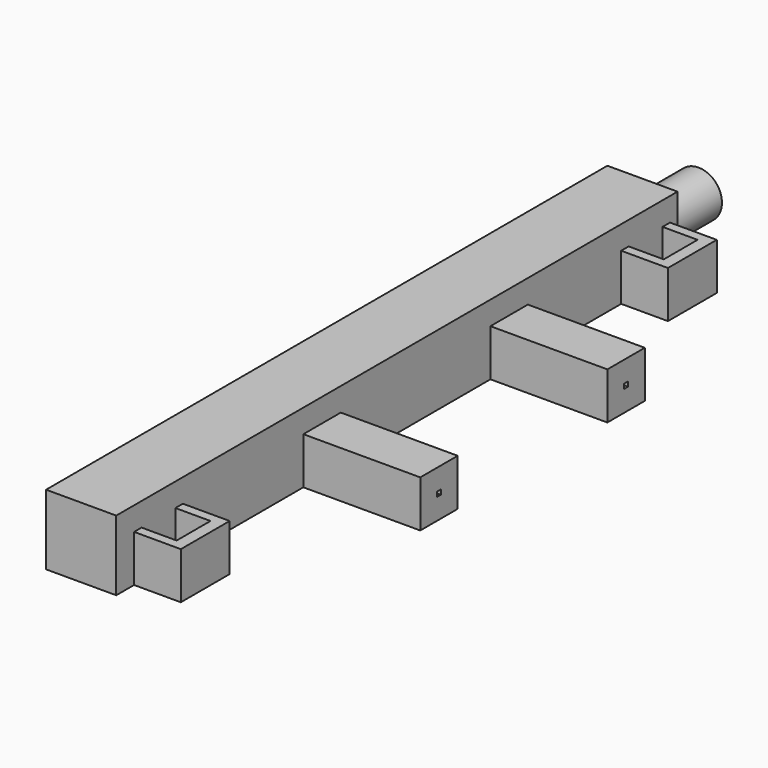
from build123d import *

# Parameters (mm, degrees)
F1_DEPTH = 15
F0_W     = 25
F0_H     = 10
F0_W_2   = 2.5
F0_H_2   = 9.0467076302
F2_DEPTH = 10
F3_W     = 4
F3_H     = 4
F4_DEPTH = 100
F6_W     = 1
F6_H     = 1
F5_W     = 1
F5_H     = 1
F7_DEPTH = 30
F8_R     = 5
F8_R_2   = 4
F9_DEPTH = 15


with BuildPart() as f1:
    # F0 (on Top) → F1 (new body)
    with BuildSketch(Plane.XY):
        Polygon((-29.806669808, 70.373563841), (-44.806669808, 70.373563841), (-44.806669808, -79.626436159), (-29.806669808, -79.626436159), (-29.806669808, -74.8653486371), (-29.806669808, -72.8653486371), (-29.806669808, -63.8186410069), (-29.806669808, -61.8186410069), (-29.806669808, -29.626436159), (-29.806669808, -19.626436159), (-29.806669808, 20.373563841), (-29.806669808, 30.373563841), (-29.806669808, 55.3112663329), (-29.806669808, 57.3112663329), (-29.806669808, 66.357973963), (-29.806669808, 68.357973963), align=None)
    extrude(amount=F1_DEPTH)

    # F0 (on Top) → F2 (join)
    with BuildSketch(Plane.XY):
        with Locations((-17.306669808, 25.373563841)):
            Rectangle(F0_W, F0_H)
        with Locations((-17.306669808, -24.626436159)):
            Rectangle(F0_W, F0_H)
        Polygon((-29.806669808, -61.8186410069), (-29.806669808, -63.8186410069), (-22.306669808, -63.8186410069), (-19.806669808, -63.8186410069), (-19.806669808, -61.8186410069), align=None)
        with Locations((-21.056669808, -68.341994822)):
            Rectangle(F0_W_2, F0_H_2)
        Polygon((-29.806669808, -72.8653486371), (-29.806669808, -74.8653486371), (-19.806669808, -74.8653486371), (-19.806669808, -72.8653486371), (-22.306669808, -72.8653486371), align=None)
        Polygon((-22.3066698015, 57.3112663329), (-29.8066698015, 57.3112663329), (-29.806669808, 55.3112663329), (-19.8066698015, 55.3112663329), (-19.8066698015, 57.3112663329), align=None)
        with Locations((-21.0566698015, 61.8346201479)):
            Rectangle(F0_W_2, F0_H_2)
        Polygon((-19.8066698015, 68.357973963), (-29.8066698015, 68.357973963), (-29.806669808, 66.357973963), (-22.3066698015, 66.357973963), (-19.8066698015, 66.357973963), align=None)
    extrude(amount=F2_DEPTH)

    # F3 (on face) → F4 (cut)
    with BuildSketch(Plane(origin=(0, 70.373563841, 0), x_dir=(-1, 0, 0), z_dir=(0, 1, 0))):
        with Locations((36.806669808, 6)):
            Rectangle(F3_W, F3_H)
    extrude(amount=-F4_DEPTH, mode=Mode.SUBTRACT)

    # F6 (on face) + F5 (on face) → F7 (cut)
    with BuildSketch(Plane.YZ.offset(-4.806669808)):
        with Locations((25.373563841, 5)):
            Rectangle(F6_W, F6_H)
    with BuildSketch(Plane.YZ.offset(-4.806669808)):
        with Locations((-24.626436159, 5)):
            Rectangle(F5_W, F5_H)
    extrude(amount=-F7_DEPTH, mode=Mode.SUBTRACT)

    # F8 (on face) → F9 (join)
    with BuildSketch(Plane(origin=(0, 70.373563841, 0), x_dir=(-1, 0, 0), z_dir=(0, 1, 0))):
        with Locations((37.306669808, 6)):
            Circle(F8_R)
        with Locations((37.306669808, 6)):
            Circle(F8_R_2, mode=Mode.SUBTRACT)
    extrude(amount=F9_DEPTH)


solid = f1.part
